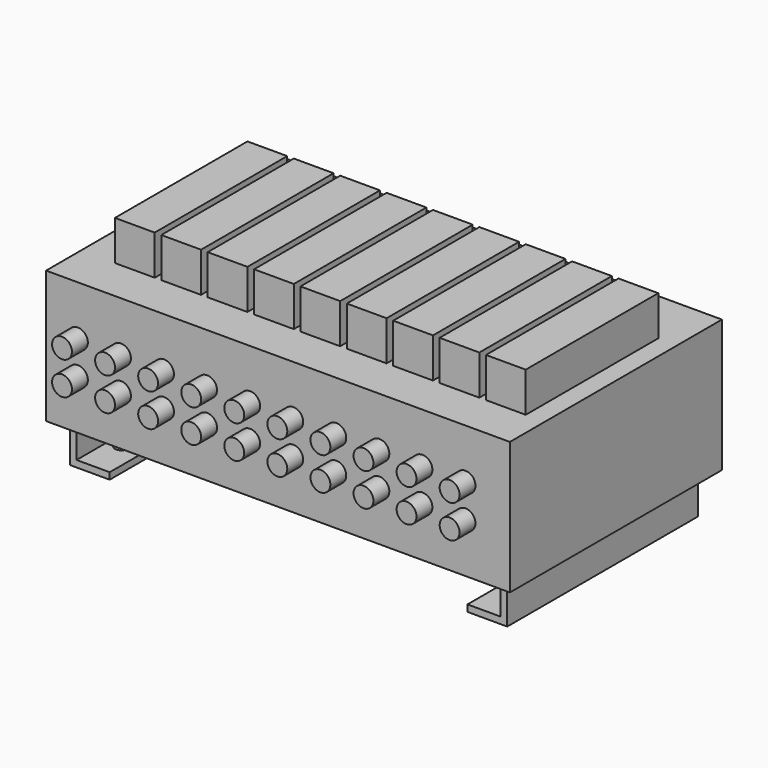
from build123d import *

# Parameters (mm, degrees)
F0_W      = 700
F0_H      = 200
F1_DEPTH  = 400
F4_DEPTH  = 360
F5_R      = 15
F6_DEPTH  = 30
F7_W      = 60
F7_H      = 250
F8_DEPTH  = 60
F9_R      = 10
F10_DEPTH = 25


# Not quite as in the source:
# - a feature names something its author has since deleted; it is built from what else it names


with BuildPart() as f1:
    # F0 (on Front) → F1 (new body)
    with BuildSketch(Plane.XZ):
        with Locations((350, 100)):
            Rectangle(F0_W, F0_H)
    extrude(amount=-F1_DEPTH)

    # F3 (on offset) → F4 (join)
    with BuildSketch(Plane.XZ.offset(-20)):
        Polygon((20, -10), (20, -19.140496552), (20, -50), (20, -60), (30, -60), (80, -60), (80, -50), (30, -50), (30, -10), (80, -10), (80, 0), (20, 0), align=None)
        Polygon((680, -10), (680, 0), (620, 0), (620, -10), (670, -10), (670, -50), (620, -50), (620, -60), (670, -60), (680, -60), align=None)
    extrude(amount=-F4_DEPTH)

    # F5 (on face) → F6 (join)
    with BuildSketch(Plane.XZ):
        with BuildLine():
            ThreePointArc((48.0253212154, 139.9992847443), (37.4187194976, 135.6058864621), (33.0253212154, 124.9992847443))
            Line((33.0253212154, 124.9992847443), (48.0253212154, 124.9992847443))
            Line((48.0253212154, 124.9992847443), (48.0253212154, 139.9992847443))
        make_face()
        with BuildLine():
            ThreePointArc((648.0253212154, 124.9992847443), (633.0253212154, 139.9992847443), (618.0253212154, 124.9992847443))
            Line((618.0253212154, 124.9992847443), (648.0253212154, 124.9992847443))
        make_face()
        with BuildLine():
            Line((648.0253212154, 124.9992847443), (618.0253212154, 124.9992847443))
            ThreePointArc((618.0253212154, 124.9992847443), (633.0253212154, 109.9992847443), (648.0253212154, 124.9992847443))
        make_face()
        with BuildLine():
            ThreePointArc((583.0253212154, 124.9992847443), (568.0253212154, 139.9992847443), (553.0253212154, 124.9992847443))
            Line((553.0253212154, 124.9992847443), (583.0253212154, 124.9992847443))
        make_face()
        with BuildLine():
            Line((583.0253212154, 124.9992847443), (553.0253212154, 124.9992847443))
            ThreePointArc((553.0253212154, 124.9992847443), (568.0253212154, 109.9992847443), (583.0253212154, 124.9992847443))
        make_face()
        with BuildLine():
            ThreePointArc((518.0253212154, 124.9992847443), (503.0253212154, 139.9992847443), (488.0253212154, 124.9992847443))
            Line((488.0253212154, 124.9992847443), (518.0253212154, 124.9992847443))
        make_face()
        with BuildLine():
            Line((518.0253212154, 124.9992847443), (488.0253212154, 124.9992847443))
            ThreePointArc((488.0253212154, 124.9992847443), (503.0253212154, 109.9992847443), (518.0253212154, 124.9992847443))
        make_face()
        with BuildLine():
            ThreePointArc((453.0253212154, 124.9992847443), (438.0253212154, 139.9992847443), (423.0253212154, 124.9992847443))
            Line((423.0253212154, 124.9992847443), (453.0253212154, 124.9992847443))
        make_face()
        with BuildLine():
            Line((453.0253212154, 124.9992847443), (423.0253212154, 124.9992847443))
            ThreePointArc((423.0253212154, 124.9992847443), (438.0253212154, 109.9992847443), (453.0253212154, 124.9992847443))
        make_face()
        with BuildLine():
            ThreePointArc((388.0253212154, 124.9992847443), (373.0253212154, 139.9992847443), (358.0253212154, 124.9992847443))
            Line((358.0253212154, 124.9992847443), (388.0253212154, 124.9992847443))
        make_face()
        with BuildLine():
            Line((388.0253212154, 124.9992847443), (358.0253212154, 124.9992847443))
            ThreePointArc((358.0253212154, 124.9992847443), (373.0253212154, 109.9992847443), (388.0253212154, 124.9992847443))
        make_face()
        with BuildLine():
            ThreePointArc((323.0253212154, 124.9992847443), (308.0253212154, 139.9992847443), (293.0253212154, 124.9992847443))
            Line((293.0253212154, 124.9992847443), (323.0253212154, 124.9992847443))
        make_face()
        with BuildLine():
            Line((323.0253212154, 124.9992847443), (293.0253212154, 124.9992847443))
            ThreePointArc((293.0253212154, 124.9992847443), (308.0253212154, 109.9992847443), (323.0253212154, 124.9992847443))
        make_face()
        with BuildLine():
            ThreePointArc((258.0253212154, 124.9992847443), (243.0253212154, 139.9992847443), (228.0253212154, 124.9992847443))
            Line((228.0253212154, 124.9992847443), (258.0253212154, 124.9992847443))
        make_face()
        with BuildLine():
            Line((258.0253212154, 124.9992847443), (228.0253212154, 124.9992847443))
            ThreePointArc((228.0253212154, 124.9992847443), (243.0253212154, 109.9992847443), (258.0253212154, 124.9992847443))
        make_face()
        with BuildLine():
            ThreePointArc((193.0253212154, 124.9992847443), (178.0253212154, 139.9992847443), (163.0253212154, 124.9992847443))
            Line((163.0253212154, 124.9992847443), (193.0253212154, 124.9992847443))
        make_face()
        with BuildLine():
            Line((193.0253212154, 124.9992847443), (163.0253212154, 124.9992847443))
            ThreePointArc((163.0253212154, 124.9992847443), (178.0253212154, 109.9992847443), (193.0253212154, 124.9992847443))
        make_face()
        with BuildLine():
            ThreePointArc((128.0253212154, 124.9992847443), (113.0253212154, 139.9992847443), (98.0253212154, 124.9992847443))
            Line((98.0253212154, 124.9992847443), (128.0253212154, 124.9992847443))
        make_face()
        with BuildLine():
            Line((128.0253212154, 124.9992847443), (98.0253212154, 124.9992847443))
            ThreePointArc((98.0253212154, 124.9992847443), (113.0253212154, 109.9992847443), (128.0253212154, 124.9992847443))
        make_face()
        with BuildLine():
            ThreePointArc((63.0253212154, 74.9992847443), (58.6319229332, 85.6058864621), (48.0253212154, 89.9992847443))
            Line((48.0253212154, 89.9992847443), (48.0253212154, 59.9992847443))
            ThreePointArc((48.0253212154, 59.9992847443), (58.6319229332, 64.3926830265), (63.0253212154, 74.9992847443))
        make_face()
        with BuildLine():
            Line((48.0253212154, 59.9992847443), (48.0253212154, 89.9992847443))
            ThreePointArc((48.0253212154, 89.9992847443), (33.0253212154, 74.9992847443), (48.0253212154, 59.9992847443))
        make_face()
        with BuildLine():
            Line((48.0253212154, 124.9992847443), (33.0253212154, 124.9992847443))
            ThreePointArc((33.0253212154, 124.9992847443), (37.4187194976, 114.3926830265), (48.0253212154, 109.9992847443))
            Line((48.0253212154, 109.9992847443), (48.0253212154, 124.9992847443))
        make_face()
        with BuildLine():
            Line((48.0253212154, 139.9992847443), (48.0253212154, 124.9992847443))
            Line((48.0253212154, 124.9992847443), (63.0253212154, 124.9992847443))
            ThreePointArc((63.0253212154, 124.9992847443), (58.6319229332, 135.6058864621), (48.0253212154, 139.9992847443))
        make_face()
        with BuildLine():
            Line((63.0253212154, 124.9992847443), (48.0253212154, 124.9992847443))
            Line((48.0253212154, 124.9992847443), (48.0253212154, 109.9992847443))
            ThreePointArc((48.0253212154, 109.9992847443), (58.6319229332, 114.3926830265), (63.0253212154, 124.9992847443))
        make_face()
        with Locations((113.0253212154, 74.9992847443)):
            Circle(F5_R)
        with Locations((178.0253212154, 74.9992847443)):
            Circle(F5_R)
        with Locations((243.0253212154, 74.9992847443)):
            Circle(F5_R)
        with Locations((308.0253212154, 74.9992847443)):
            Circle(F5_R)
        with Locations((373.0253212154, 74.9992847443)):
            Circle(F5_R)
        with Locations((438.0253212154, 74.9992847443)):
            Circle(F5_R)
        with Locations((503.0253212154, 74.9992847443)):
            Circle(F5_R)
        with Locations((568.0253212154, 74.9992847443)):
            Circle(F5_R)
        with Locations((633.0253212154, 74.9992847443)):
            Circle(F5_R)
    extrude(amount=F6_DEPTH)

    # F7 (on face) → F8 (join)
    with BuildSketch(Plane.XY.offset(200)):
        with Locations((81.3367652893, 190.7173022628)):
            Rectangle(F7_W, F7_H)
        with Locations((151.3367652893, 190.7173022628)):
            Rectangle(F7_W, F7_H)
        with Locations((221.3367652893, 190.7173022628)):
            Rectangle(F7_W, F7_H)
        with Locations((291.3367652893, 190.7173022628)):
            Rectangle(F7_W, F7_H)
        with Locations((361.3367652893, 190.7173022628)):
            Rectangle(F7_W, F7_H)
        with Locations((431.3367652893, 190.7173022628)):
            Rectangle(F7_W, F7_H)
        with Locations((501.3367652893, 190.7173022628)):
            Rectangle(F7_W, F7_H)
        with Locations((571.3367652893, 190.7173022628)):
            Rectangle(F7_W, F7_H)
        with Locations((641.3367652893, 190.7173022628)):
            Rectangle(F7_W, F7_H)
    extrude(amount=F8_DEPTH)

    # F9 (on face) → F10 (cut)
    with BuildSketch(Plane(origin=(0, 0, -60), x_dir=(1, 0, 0), z_dir=(0, 0, -1))):
        with BuildLine():
            ThreePointArc((50, -310), (40, -320), (50, -330))
            Line((50, -330), (50, -310))
        make_face()
        with BuildLine():
            ThreePointArc((50, -70), (40, -80), (50, -90))
            Line((50, -90), (50, -70))
        make_face()
        with BuildLine():
            Line((50, -70), (50, -90))
            ThreePointArc((50, -90), (57.0710678119, -87.0710678119), (60, -80))
            ThreePointArc((60, -80), (57.0710678119, -72.9289321881), (50, -70))
        make_face()
        with BuildLine():
            Line((50, -310), (50, -330))
            ThreePointArc((50, -330), (57.0710678119, -327.0710678119), (60, -320))
            ThreePointArc((60, -320), (57.0710678119, -312.9289321881), (50, -310))
        make_face()
        with Locations((650.3430891037, -320)):
            Circle(F9_R)
        with Locations((650.3430891037, -80)):
            Circle(F9_R)
    extrude(amount=-F10_DEPTH, mode=Mode.SUBTRACT)


solid = f1.part
